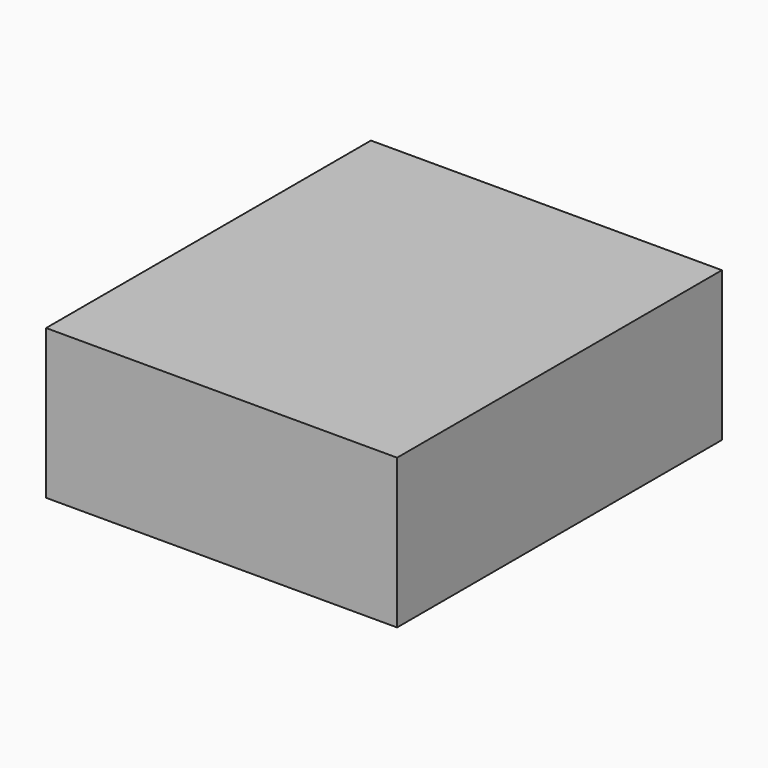
from build123d import *

# Parameters (mm, degrees)
F0_W     = 83.9887112379
F0_H     = 35.7687845826
F1_DEPTH = 97.1562061459


# Not quite as in the source:
# - the program builds the solid bodies; features that only make, move or delete a surface that nothing else refers to are left out


with BuildPart() as f1:
    # F0 (on Front) → F1 (new body)
    with BuildSketch(Plane.XZ):
        with Locations((1.2451484799, 9.9609233439)):
            Rectangle(F0_W, F0_H)
    extrude(amount=F1_DEPTH)


solid = f1.part
